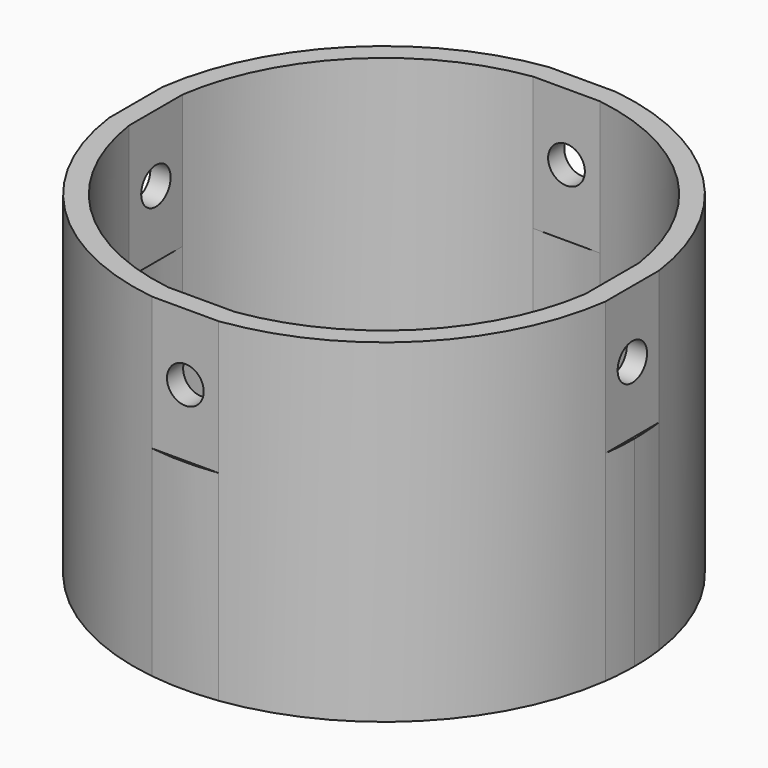
from build123d import *

# Parameters (mm, degrees)
F1_DEPTH = 20
F3_D     = 5.5
F5_D     = 5.5
F7_DEPTH = 30


# Not quite as in the source:
# - after a boolean that leaves OpenCascade's solid faulty, fix() repairs it


with BuildPart() as f1:
    # F0 (on Top) → F1 (new body)
    with BuildSketch(Plane.XY):
        with BuildLine():
            Line((37.1651718683, -5), (37.1651718683, 5))
            ThreePointArc((37.1651718683, 5), (26.5165042945, 26.5165042945), (5, 37.1651718683))
            Line((5, 37.1651718683), (-5, 37.1651718683))
            ThreePointArc((-5, 37.1651718683), (-26.5165042945, 26.5165042945), (-37.1651718683, 5))
            Line((-37.1651718683, 5), (-37.1651718683, -5))
            ThreePointArc((-37.1651718683, -5), (-26.5165042945, -26.5165042945), (-5, -37.1651718683))
            Line((-5, -37.1651718683), (5, -37.1651718683))
            ThreePointArc((5, -37.1651718683), (26.5165042945, -26.5165042945), (37.1651718683, -5))
        make_face()
        with BuildLine():
            ThreePointArc((-5, -34.1357583774), (-24.3951839509, -24.3951839509), (-34.1357583774, -5))
            Line((-34.1357583774, -5), (-34.1357583774, 5))
            ThreePointArc((-34.1357583774, 5), (-24.3951839509, 24.3951839509), (-5, 34.1357583774))
            Line((-5, 34.1357583774), (5, 34.1357583774))
            ThreePointArc((5, 34.1357583774), (24.3951839509, 24.3951839509), (34.1357583774, 5))
            Line((34.1357583774, 5), (34.1357583774, -5))
            ThreePointArc((34.1357583774, -5), (24.3951839509, -24.3951839509), (5, -34.1357583774))
            Line((5, -34.1357583774), (-5, -34.1357583774))
        make_face(mode=Mode.SUBTRACT)
    extrude(amount=F1_DEPTH)

    # F3 (through all)
    with Locations(Plane.YZ.offset(37.1651718683)):
        with Locations((0, 10)):
            Hole(F3_D / 2)

    # F5 (through all)
    with Locations(Plane.XZ.offset(37.1651718683)):
        with Locations((0, 10)):
            Hole(F5_D / 2)

    # F6 (on face) → F7 (join)
    with BuildSketch(Plane(origin=(0, 0, 0), x_dir=(1, 0, 0), z_dir=(0, 0, -1))):
        with BuildLine():
            Line((37.1651718683, -5), (37.1651718683, 5))
            ThreePointArc((37.1651718683, 5), (26.5165042945, 26.5165042945), (5, 37.1651718683))
            Line((5, 37.1651718683), (-5, 37.1651718683))
            ThreePointArc((-5, 37.1651718683), (-26.5165042945, 26.5165042945), (-37.1651718683, 5))
            Line((-37.1651718683, 5), (-37.1651718683, -5))
            ThreePointArc((-37.1651718683, -5), (-26.5165042945, -26.5165042945), (-5, -37.1651718683))
            Line((-5, -37.1651718683), (5, -37.1651718683))
            ThreePointArc((5, -37.1651718683), (26.5165042945, -26.5165042945), (37.1651718683, -5))
        make_face()
        with BuildLine():
            ThreePointArc((34.1357583774, 5), (34.4088191022, 2.5066248203), (34.5, 0))
            ThreePointArc((34.5, 0), (34.4088191022, -2.5066248203), (34.1357583774, -5))
            ThreePointArc((34.1357583774, -5), (24.3951839509, -24.3951839509), (5, -34.1357583774))
            ThreePointArc((5, -34.1357583774), (0, -34.5), (-5, -34.1357583774))
            ThreePointArc((-5, -34.1357583774), (-24.3951839509, -24.3951839509), (-34.1357583774, -5))
            ThreePointArc((-34.1357583774, -5), (-34.5, 0), (-34.1357583774, 5))
            ThreePointArc((-34.1357583774, 5), (-24.3951839509, 24.3951839509), (-5, 34.1357583774))
            ThreePointArc((-5, 34.1357583774), (0, 34.5), (5, 34.1357583774))
            ThreePointArc((5, 34.1357583774), (24.3951839509, 24.3951839509), (34.1357583774, 5))
        make_face(mode=Mode.SUBTRACT)
        with BuildLine():
            Line((-5, 37.1651718683), (5, 37.1651718683))
            ThreePointArc((5, 37.1651718683), (0, 37.5), (-5, 37.1651718683))
        make_face()
        with BuildLine():
            ThreePointArc((37.1651718683, -5), (37.4161993331, -2.5055992236), (37.5, 0))
            ThreePointArc((37.5, 0), (37.4161993331, 2.5055992236), (37.1651718683, 5))
            Line((37.1651718683, 5), (37.1651718683, -5))
        make_face()
        with BuildLine():
            ThreePointArc((-5, -37.1651718683), (0, -37.5), (5, -37.1651718683))
            Line((5, -37.1651718683), (-5, -37.1651718683))
        make_face()
        with BuildLine():
            Line((-37.1651718683, -5), (-37.1651718683, 5))
            ThreePointArc((-37.1651718683, 5), (-37.5, 0), (-37.1651718683, -5))
        make_face()
    extrude(amount=F7_DEPTH)

    add(f1.part.fix(), mode=Mode.REPLACE)


solid = f1.part
